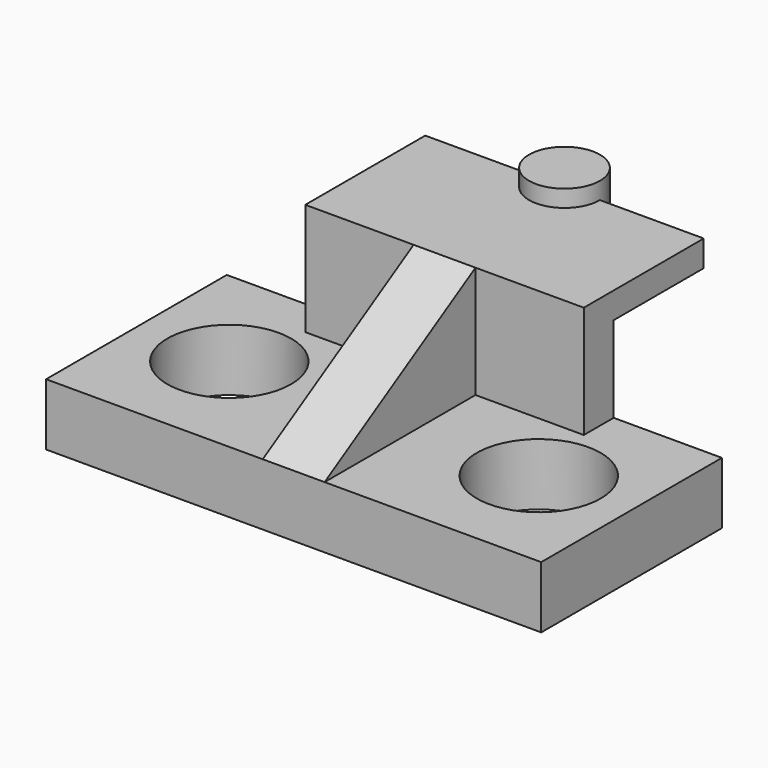
from build123d import *

# Parameters (mm, degrees)
F1_DEPTH = 101.6
F2_DEPTH = 12.7
F3_DEPTH = 57.15
F0_W     = 14.5453011187
F0_H     = 10.745606224
F4_DEPTH = 57.15
F6_R     = 25.4
F7_DEPTH = 12.7


# Not quite as in the source:
# - a feature names something its author has since deleted; it is built from what else it names


with BuildPart() as f1:
    # F0 (on Right) → F1 (new body, symmetric)
    with BuildSketch(Plane.YZ):
        Polygon((31.0628309338, 12.7), (-46.3495767937, 12.7), (-46.3495767937, -12.7), (46.3495767937, -12.7), (46.3495767937, 12.7), align=None)
    extrude(amount=F1_DEPTH, both=True)

    # F0 (on Right) → F2 (join, symmetric)
    with BuildSketch(Plane.YZ):
        Polygon((31.0628309338, 58.703106785), (-46.3495767937, 12.7), (31.0628309338, 12.7), align=None)
    extrude(amount=F2_DEPTH, both=True)

    # F0 (on Right) → F3 (join, symmetric)
    with BuildSketch(Plane.YZ):
        Polygon((31.0628309338, 58.703106785), (31.0628309338, 12.7), (46.3495767937, 12.7), (46.3495767937, 47.9575005611), (78.0453036841, 47.9575005611), (78.0453036841, 58.703106785), align=None)
    extrude(amount=F3_DEPTH, both=True)

    # F0 (on Right) → F4 (join, symmetric)
    with BuildSketch(Plane.YZ):
        with Locations((85.3179542435, 53.330303673)):
            Rectangle(F0_W, F0_H)
    extrude(amount=F4_DEPTH, both=True)

    # F0 (on Right) → F5 (revolve)
    with BuildSketch(Plane.YZ):
        Polygon((92.5906048029, 65.6709397763), (92.5906048029, 58.703106785), (92.5906048029, 47.9575005611), (92.5906048029, 36.5803426697), (107.1359059216, 36.5803426697), (107.1359059216, 65.6709397763), align=None)
    revolve(axis=Axis((0, 92.5906048029, 51.125641223), (0, 0, -1)))

    # F6 (on Top) → F7 (cut, symmetric)
    with BuildSketch(Plane.XY):
        with Locations((-63.5, 0)):
            Circle(F6_R)
        with Locations((63.5, 0)):
            Circle(F6_R)
    extrude(amount=F7_DEPTH, both=True, mode=Mode.SUBTRACT)


solid = f1.part
